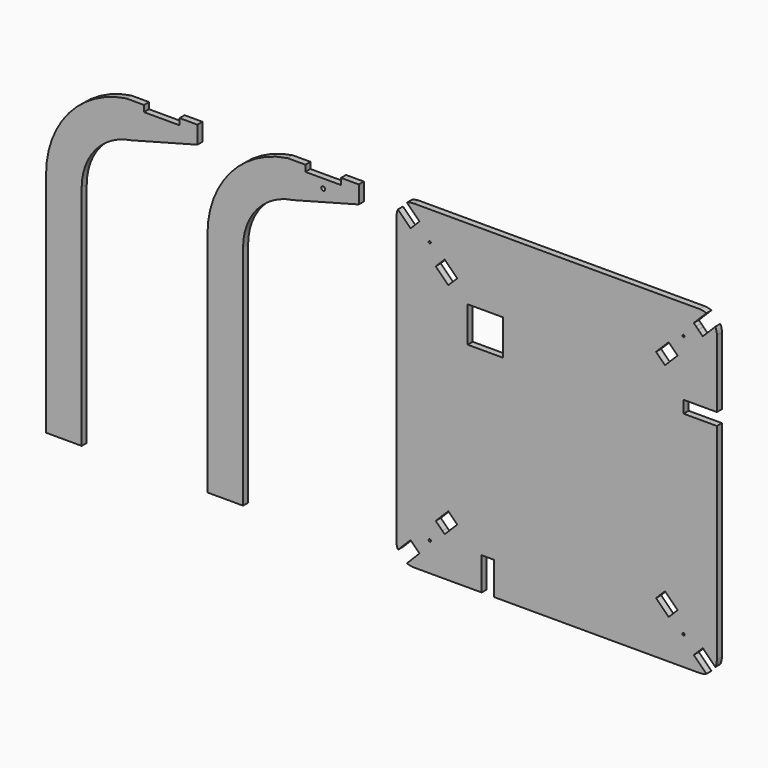
from build123d import *

# Parameters (mm, degrees)
F0_R     = 5.588
F1_DEPTH = 18.034
F0_W     = 101.6
F0_H     = 101.6
F0_R_2   = 3.175


# Not quite as in the source:
# - a feature names something its author has since deleted; it is built from what else it names


with BuildPart() as f1:
    # F0 (on Front) → F1 (new body)
    with BuildSketch(Plane.XZ):
        with BuildLine():
            Line((483.2065144254, 424.6733268274), (432.4065144254, 424.6733268274))
            ThreePointArc((432.4065144254, 424.6733268274), (268.8463203697, 334.5643709124), (203.8065144254, 159.5175638624))
            Line((203.8065144254, 159.5175638624), (203.8065144254, -489.7266731726))
            Line((203.8065144254, -489.7266731726), (305.4065144254, -489.7266731726))
            Line((305.4065144254, -489.7266731726), (305.4065144254, 159.5175638624))
            ThreePointArc((305.4065144254, 159.5175638624), (345.7966685973, 268.2228009306), (447.3686422275, 324.1810647789))
            Line((447.3686422275, 324.1810647789), (635.6065144254, 374.3450939655))
            Line((635.6065144254, 374.3450939655), (635.6065144254, 406.6393268274))
            Line((635.6065144254, 406.6393268274), (635.6065144254, 424.6733268274))
            Line((635.6065144254, 424.6733268274), (584.8065144254, 424.6733268274))
            Line((584.8065144254, 424.6733268274), (584.8065144254, 406.6393268274))
            Line((584.8065144254, 406.6393268274), (483.2065144254, 406.6393268274))
            Line((483.2065144254, 406.6393268274), (483.2065144254, 424.6733268274))
        make_face()
        with Locations((534.0065144254, 381.2393268274)):
            Circle(F0_R, mode=Mode.SUBTRACT)
    extrude(amount=F1_DEPTH)


with BuildPart() as f1b:
    # F0 (on Front) → F1, piece 2 (new body)
    with BuildSketch(Plane.XZ):
        with BuildLine():
            Line((1607.6519874032, 427.9213663064), (792.8783607687, 427.9213663064))
            ThreePointArc((792.8783607687, 427.9213663064), (782.6863062078, 426.8675437634), (772.9254875333, 423.7506644064))
            Line((772.9254875333, 423.7506644064), (808.7447410617, 387.7281564889))
            Line((808.7447410617, 387.7281564889), (795.956750751, 375.0123214863))
            Line((795.956750751, 375.0123214863), (783.1687604403, 362.2964864837))
            Line((783.1687604403, 362.2964864837), (747.3495069119, 398.3189944012))
            ThreePointArc((747.3495069119, 398.3189944012), (744.1480269708, 388.4381426165), (743.0651740859, 378.1081796236))
            Line((743.0651740859, 378.1081796236), (743.0651740859, -436.6654470109))
            ThreePointArc((743.0651740859, -436.6654470109), (744.1480269708, -446.9954100037), (747.3495069119, -456.8762617884))
            Line((747.3495069118, -456.8762617884), (783.1687604403, -420.8537538709))
            Line((783.1687604403, -420.8537538709), (795.956750751, -433.5695888735))
            Line((795.956750751, -433.5695888735), (802.3507459063, -439.9275063748))
            Line((802.3507459063, -439.9275063748), (808.7447410617, -446.2854238761))
            Line((808.7447410617, -446.2854238761), (772.9254875333, -482.3079317936))
            ThreePointArc((772.9254875333, -482.3079317936), (782.6863062078, -485.4248111507), (792.8783607687, -486.4786336936))
            Line((792.8783607687, -486.4786336936), (986.2313252449, -486.4786336936))
            Line((986.2313252449, -486.4786336936), (986.2313252449, -392.7684829235))
            Line((986.2313252449, -392.7684829235), (1021.1563252449, -392.7684829235))
            Line((1021.1563252449, -392.7684829235), (1021.1563252449, -486.4786336936))
            Line((1021.1563252449, -486.4786336936), (1607.6519874032, -486.4786336936))
            ThreePointArc((1607.6519874032, -486.4786336936), (1617.8440419641, -485.4248111507), (1627.6048606386, -482.3079317936))
            Line((1627.6048606386, -482.3079317936), (1591.7856071102, -446.2854238761))
            Line((1591.7856071102, -446.2854238761), (1598.1796022655, -439.9275063748))
            Line((1598.1796022655, -439.9275063748), (1604.5735974209, -433.5695888735))
            Line((1604.5735974209, -433.5695888735), (1617.3615877316, -420.8537538709))
            Line((1617.3615877316, -420.8537538709), (1653.18084126, -456.8762617884))
            ThreePointArc((1653.18084126, -456.8762617884), (1656.3823212011, -446.9954100037), (1657.4651740859, -436.6654470109))
            Line((1657.4651740859, -436.6654470109), (1657.4651740859, 150.1565170765))
            Line((1657.4651740859, 150.1565170765), (1562.2151740859, 150.1565170765))
            Line((1562.2151740859, 150.1565170765), (1562.2151740859, 185.0815170765))
            Line((1562.2151740859, 185.0815170765), (1657.4651740859, 185.0815170765))
            Line((1657.4651740859, 185.0815170765), (1657.4651740859, 378.1081796236))
            ThreePointArc((1657.4651740859, 378.1081796236), (1656.3823212011, 388.4381426165), (1653.18084126, 398.3189944012))
            Line((1653.18084126, 398.3189944012), (1617.3615877316, 362.2964864837))
            Line((1617.3615877316, 362.2964864837), (1604.5735974209, 375.0123214863))
            Line((1604.5735974209, 375.0123214863), (1598.1796022655, 381.3702389876))
            Line((1598.1796022655, 381.3702389876), (1591.7856071102, 387.7281564889))
            Line((1591.7856071102, 387.7281564889), (1627.6048606386, 423.7506644064))
            ThreePointArc((1627.6048606386, 423.7506644064), (1617.8440419641, 426.8675437634), (1607.6519874032, 427.9213663064))
        make_face()
        with BuildLine():
            ThreePointArc((841.3632739356, -403.8866202588), (839.4074420696, -406.8182160804), (835.9495705901, -406.1380270037))
            ThreePointArc((835.9495705901, -406.1380270037), (835.0132810832, -403.8933572576), (835.9400362986, -401.6447343278))
            ThreePointArc((835.9400362986, -401.6447343278), (838.1815369368, -400.7116274064), (840.4269772811, -401.635213514))
            ThreePointArc((840.4269772811, -401.635213514), (841.1198697572, -402.6674521248), (841.3632739356, -403.8866202588))
        make_face(mode=Mode.SUBTRACT)
        Polygon((880.6885609861, -374.5448583408), (874.0076708186, -367.8639681733), (855.1846336023, -349.0409309569), (891.1056580866, -313.1199064727), (916.6095854704, -338.6238338565), align=None, mode=Mode.SUBTRACT)
        with BuildLine():
            ThreePointArc((1565.5170742363, -403.8866202588), (1565.2736700579, -405.1057883928), (1564.5807775818, -406.1380270037))
            ThreePointArc((1564.5807775818, -406.1380270037), (1560.0906674915, -406.1253236043), (1560.1033708908, -401.635213514))
            ThreePointArc((1560.1033708908, -401.635213514), (1562.3488112351, -400.7116274064), (1564.5903118733, -401.6447343278))
            ThreePointArc((1564.5903118733, -401.6447343278), (1565.2762503981, -402.6736753915), (1565.5170742363, -403.8866202588))
        make_face(mode=Mode.SUBTRACT)
        Polygon((1545.3457145696, -349.0409309569), (1526.5226773533, -367.8639681733), (1519.8417871858, -374.5448583408), (1483.9207627015, -338.6238338565), (1509.4246900853, -313.1199064727), align=None, mode=Mode.SUBTRACT)
        with Locations((997.0651740859, 173.9213663064)):
            Rectangle(F0_W, F0_H, mode=Mode.SUBTRACT)
        Polygon((891.1056580866, 254.5626390854), (855.1846336023, 290.4836635697), (880.6885609861, 315.9875909535), (916.6095854704, 280.0665664693), align=None, mode=Mode.SUBTRACT)
        with Locations((838.1882739356, 345.3293528716)):
            Circle(F0_R_2, mode=Mode.SUBTRACT)
        Polygon((1519.8417871858, 315.9875909535), (1526.5226773533, 309.306700786), (1545.3457145696, 290.4836635697), (1509.4246900853, 254.5626390854), (1483.9207627015, 280.0665664693), align=None, mode=Mode.SUBTRACT)
        with BuildLine():
            ThreePointArc((1560.1033708908, 343.0779461267), (1560.0906674915, 347.5680562171), (1564.5807775818, 347.5807596164))
            ThreePointArc((1564.5807775818, 347.5807596164), (1565.2736700579, 346.5485210056), (1565.5170742363, 345.3293528716))
            ThreePointArc((1565.5170742363, 345.3293528716), (1565.2762503981, 344.1164080042), (1564.5903118733, 343.0874669406))
            ThreePointArc((1564.5903118733, 343.0874669406), (1562.3488112351, 342.1543600192), (1560.1033708908, 343.0779461267))
        make_face(mode=Mode.SUBTRACT)
    extrude(amount=F1_DEPTH)


with BuildPart() as f1c:
    # F0 (on Front) → F1, piece 3 (new body)
    with BuildSketch(Plane.XZ):
        with BuildLine():
            Line((-256.7524378796, 159.8593657013), (-256.7524378796, -489.3848713337))
            Line((-256.7524378796, -489.3848713337), (-155.1524378796, -489.3848713337))
            Line((-155.1524378796, -489.3848713337), (-155.1524378796, 159.8593657013))
            ThreePointArc((-155.1524378796, 159.8593657013), (-114.7622837077, 268.5646027694), (-13.1903100775, 324.5228666178))
            Line((-13.1903100775, 324.5228666178), (175.0475621204, 374.6868958044))
            Line((175.0475621204, 374.6868958044), (175.0475621204, 406.9811286663))
            Line((175.0475621204, 406.9811286663), (175.0475621204, 425.0151286663))
            Line((175.0475621204, 425.0151286663), (124.2475621204, 425.0151286663))
            Line((124.2475621204, 425.0151286663), (124.2475621204, 406.9811286663))
            Line((124.2475621204, 406.9811286663), (22.6475621204, 406.9811286663))
            Line((22.6475621204, 406.9811286663), (22.6475621204, 425.0151286663))
            Line((22.6475621204, 425.0151286663), (-28.1524378796, 425.0151286663))
            ThreePointArc((-28.1524378796, 425.0151286663), (-191.7126319353, 334.9061727512), (-256.7524378796, 159.8593657013))
        make_face()
    extrude(amount=F1_DEPTH)


solid = Compound([f1.part, f1b.part, f1c.part])
